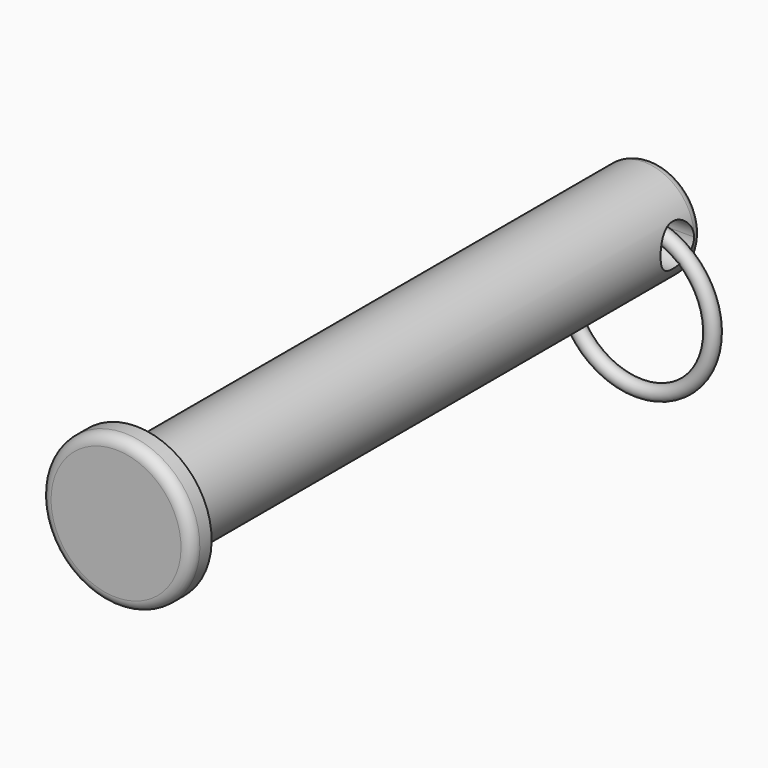
from build123d import *

# Parameters (mm, degrees)
F2_R     = 1
F3_DEPTH = 12.5
F4_R     = 0.49999
F5_R     = 0.35


# Not quite as in the source:
# - a fillet or chamfer is up to 0.001 mm smaller than in the source, because OpenCascade refuses the exact size


with BuildPart() as f1:
    # F0 (on Right) → F1 (revolve)
    with BuildSketch(Plane.YZ):
        Polygon((-1.2, 3.6), (-1.2, 0), (30.8, 0), (30.8, 2.38), (0, 2.38), (0, 3.6), align=None)
    revolve(axis=Axis((0, 14.8, 0), (0, -1, 0)))

    # F2 (on Right) → F3 (cut, symmetric)
    with BuildSketch(Plane.YZ):
        with Locations((29.3, 0)):
            Circle(F2_R)
    extrude(amount=F3_DEPTH, both=True, mode=Mode.SUBTRACT)

    # F4 (radius 0.5 in the source; OpenCascade refuses exactly that, so slightly less here)
    f4_edges = [f1.edges().sort_by_distance(p)[0] for p in [
        (0, -1.2, -3.6),
        (0, 30.8, -2.38),
    ]]
    fillet(f4_edges, radius=F4_R)

    # F5 (on Right) → F6 (revolve)
    with BuildSketch(Plane.YZ):
        with Locations((30, 0)):
            Circle(F5_R)
    revolve(axis=Axis((0, 28.3114453778, -3.5), (0, 1, 0)))


solid = f1.part
